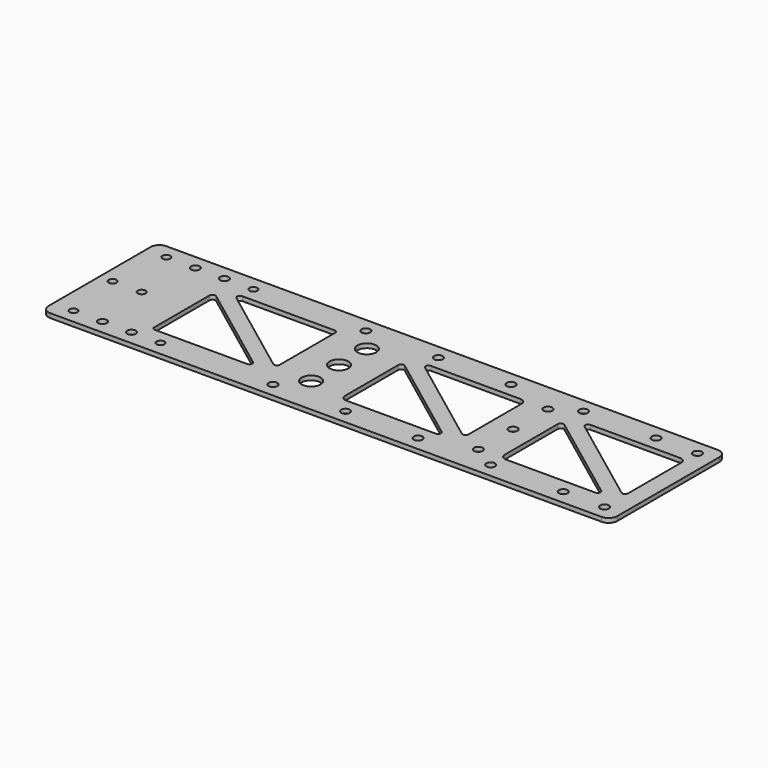
from build123d import *

# Parameters (mm, degrees)
F0_R     = 3.25
F0_R_2   = 1.35
F0_R_3   = 1.5
F1_DEPTH = 1.5


# Not quite as in the source:
# - a feature names something its author has since deleted; it is built from what else it names


with BuildPart() as f1:
    # F0 (on Top) → F1 (new body)
    with BuildSketch(Plane.XY):
        with BuildLine():
            Line((61.8890674149, 727.822291851), (-128.1109325851, 727.822291851))
            ThreePointArc((-128.1109325851, 727.822291851), (-130.2322529287, 726.9436121946), (-131.1109325851, 724.822291851))
            Line((-131.1109325851, 724.822291851), (-131.1109325851, 702.822291851))
            Line((-131.1109325851, 702.822291851), (-127.9609325851, 702.822291851))
            ThreePointArc((-127.9609325851, 702.822291851), (-126.6109325851, 704.172291851), (-125.2609325851, 702.822291851))
            Line((-125.2609325851, 702.822291851), (-117.9609325851, 702.822291851))
            ThreePointArc((-117.9609325851, 702.822291851), (-116.6109325851, 704.172291851), (-115.2609325851, 702.822291851))
            Line((-115.2609325851, 702.822291851), (-101.1109325851, 702.822291851))
            Line((-101.1109325851, 702.822291851), (-101.1109325851, 712.697291851))
            Line((-101.1109325851, 712.697291851), (-101.1109325851, 714.697291851))
            Line((-101.1109325851, 714.697291851), (-101.1109325851, 714.822291851))
            ThreePointArc((-101.1109325851, 714.822291851), (-100.8472193445, 716.0522246827), (-100.1024427382, 717.0659244658))
            ThreePointArc((-100.1024427382, 717.0659244658), (-99.1760856623, 717.6268326195), (-98.1109325851, 717.822291851))
            Line((-98.1109325851, 717.822291851), (-96.9442659185, 717.822291851))
            Line((-96.9442659185, 717.822291851), (-93.9442659185, 717.822291851))
            Line((-93.9442659185, 717.822291851), (-62.1109325851, 717.822291851))
            ThreePointArc((-62.1109325851, 717.822291851), (-61.403825804, 717.5293986322), (-61.1109325851, 716.822291851))
            Line((-61.1109325851, 716.822291851), (-61.1109325851, 702.822291851))
            Line((-61.1109325851, 702.822291851), (-51.8609325851, 702.822291851))
            ThreePointArc((-51.8609325851, 702.822291851), (-48.6109325851, 706.072291851), (-45.3609325851, 702.822291851))
            Line((-45.3609325851, 702.822291851), (-36.1109325851, 702.822291851))
            Line((-36.1109325851, 702.822291851), (-36.1109325851, 712.697291851))
            Line((-36.1109325851, 712.697291851), (-36.1109325851, 714.697291851))
            Line((-36.1109325851, 714.697291851), (-36.1109325851, 715.822291851))
            ThreePointArc((-36.1109325851, 715.822291851), (-35.9351237581, 716.6422470721), (-35.4386060205, 717.3180469276))
            ThreePointArc((-35.4386060205, 717.3180469276), (-34.8210346366, 717.6919856967), (-34.1109325851, 717.822291851))
            Line((-34.1109325851, 717.822291851), (-31.9442659185, 717.822291851))
            Line((-31.9442659185, 717.822291851), (-28.9442659185, 717.822291851))
            Line((-28.9442659185, 717.822291851), (1.8890674149, 717.822291851))
            ThreePointArc((1.8890674149, 717.822291851), (3.3032809772, 717.2365054134), (3.8890674149, 715.822291851))
            Line((3.8890674149, 715.822291851), (3.8890674149, 702.822291851))
            Line((3.8890674149, 702.822291851), (9.8890674149, 702.822291851))
            ThreePointArc((9.8890674149, 702.822291851), (11.3890674149, 704.322291851), (12.8890674149, 702.822291851))
            Line((12.8890674149, 702.822291851), (18.8890674149, 702.822291851))
            Line((18.8890674149, 702.822291851), (18.8890674149, 712.697291851))
            Line((18.8890674149, 712.697291851), (18.8890674149, 714.697291851))
            Line((18.8890674149, 714.697291851), (18.8890674149, 715.822291851))
            ThreePointArc((18.8890674149, 715.822291851), (19.0648762419, 716.6422470721), (19.5613939795, 717.3180469276))
            ThreePointArc((19.5613939795, 717.3180469276), (20.1789653634, 717.6919856967), (20.8890674149, 717.822291851))
            Line((20.8890674149, 717.822291851), (23.0557340815, 717.822291851))
            Line((23.0557340815, 717.822291851), (26.0557340815, 717.822291851))
            Line((26.0557340815, 717.822291851), (56.8890674149, 717.822291851))
            ThreePointArc((56.8890674149, 717.822291851), (58.3032809772, 717.2365054134), (58.8890674149, 715.822291851))
            Line((58.8890674149, 715.822291851), (58.8890674149, 702.822291851))
            Line((58.8890674149, 702.822291851), (64.8890674149, 702.822291851))
            Line((64.8890674149, 702.822291851), (64.8890674149, 724.822291851))
            ThreePointArc((64.8890674149, 724.822291851), (64.0103877584, 726.9436121946), (61.8890674149, 727.822291851))
        make_face()
        with Locations((-48.6109325851, 714.822291851)):
            Circle(F0_R, mode=Mode.SUBTRACT)
        with Locations((-124.1109325851, 722.822291851)):
            Circle(F0_R_2, mode=Mode.SUBTRACT)
        with Locations((-114.1109325851, 722.822291851)):
            Circle(F0_R_3, mode=Mode.SUBTRACT)
        with Locations((-104.1109325851, 722.822291851)):
            Circle(F0_R_3, mode=Mode.SUBTRACT)
        with Locations((-94.1109325851, 722.822291851)):
            Circle(F0_R_2, mode=Mode.SUBTRACT)
        with Locations((-55.3609325851, 722.822291851)):
            Circle(F0_R_3, mode=Mode.SUBTRACT)
        with Locations((11.3890674149, 717.822291851)):
            Circle(F0_R_3, mode=Mode.SUBTRACT)
        with Locations((-30.3609325851, 722.822291851)):
            Circle(F0_R_3, mode=Mode.SUBTRACT)
        with Locations((-5.3609325851, 722.822291851)):
            Circle(F0_R_3, mode=Mode.SUBTRACT)
        with Locations((19.6390674149, 722.822291851)):
            Circle(F0_R_3, mode=Mode.SUBTRACT)
        with Locations((23.8890674149, 722.822291851)):
            Circle(F0_R_3, mode=Mode.SUBTRACT)
        with Locations((44.6390674149, 722.822291851)):
            Circle(F0_R_3, mode=Mode.SUBTRACT)
        with Locations((58.8890674149, 722.822291851)):
            Circle(F0_R_3, mode=Mode.SUBTRACT)
        with BuildLine():
            Line((-127.9609325851, 702.822291851), (-131.1109325851, 702.822291851))
            Line((-131.1109325851, 702.822291851), (-131.1109325851, 680.822291851))
            ThreePointArc((-131.1109325851, 680.822291851), (-130.2322529287, 678.7009715075), (-128.1109325851, 677.822291851))
            Line((-128.1109325851, 677.822291851), (61.8890674149, 677.822291851))
            ThreePointArc((61.8890674149, 677.822291851), (64.0103877584, 678.7009715075), (64.8890674149, 680.822291851))
            Line((64.8890674149, 680.822291851), (64.8890674149, 702.822291851))
            Line((64.8890674149, 702.822291851), (58.8890674149, 702.822291851))
            Line((58.8890674149, 702.822291851), (58.8890674149, 692.947291851))
            Line((58.8890674149, 692.947291851), (58.8890674149, 690.947291851))
            Line((58.8890674149, 690.947291851), (58.8890674149, 689.822291851))
            ThreePointArc((58.8890674149, 689.822291851), (58.7132585878, 689.0023366299), (58.2167408502, 688.3265367745))
            ThreePointArc((58.2167408502, 688.3265367745), (57.5991694663, 687.9525980054), (56.8890674149, 687.822291851))
            Line((56.8890674149, 687.822291851), (54.7224007482, 687.822291851))
            Line((54.7224007482, 687.822291851), (51.7224007482, 687.822291851))
            Line((51.7224007482, 687.822291851), (20.8890674149, 687.822291851))
            ThreePointArc((20.8890674149, 687.822291851), (19.4748538525, 688.4080782887), (18.8890674149, 689.822291851))
            Line((18.8890674149, 689.822291851), (18.8890674149, 702.822291851))
            Line((18.8890674149, 702.822291851), (12.8890674149, 702.822291851))
            ThreePointArc((12.8890674149, 702.822291851), (11.3890674149, 701.322291851), (9.8890674149, 702.822291851))
            Line((9.8890674149, 702.822291851), (3.8890674149, 702.822291851))
            Line((3.8890674149, 702.822291851), (3.8890674149, 692.947291851))
            Line((3.8890674149, 692.947291851), (3.8890674149, 690.947291851))
            Line((3.8890674149, 690.947291851), (3.8890674149, 689.822291851))
            ThreePointArc((3.8890674149, 689.822291851), (3.7132585878, 689.0023366299), (3.2167408502, 688.3265367745))
            ThreePointArc((3.2167408502, 688.3265367745), (2.5991694663, 687.9525980054), (1.8890674149, 687.822291851))
            Line((1.8890674149, 687.822291851), (-0.2775992518, 687.822291851))
            Line((-0.2775992518, 687.822291851), (-3.2775992518, 687.822291851))
            Line((-3.2775992518, 687.822291851), (-34.1109325851, 687.822291851))
            ThreePointArc((-34.1109325851, 687.822291851), (-35.5251461475, 688.4080782887), (-36.1109325851, 689.822291851))
            Line((-36.1109325851, 689.822291851), (-36.1109325851, 702.822291851))
            Line((-36.1109325851, 702.822291851), (-45.3609325851, 702.822291851))
            ThreePointArc((-45.3609325851, 702.822291851), (-48.6109325851, 699.572291851), (-51.8609325851, 702.822291851))
            Line((-51.8609325851, 702.822291851), (-61.1109325851, 702.822291851))
            Line((-61.1109325851, 702.822291851), (-61.1109325851, 692.947291851))
            Line((-61.1109325851, 692.947291851), (-61.1109325851, 690.947291851))
            Line((-61.1109325851, 690.947291851), (-61.1109325851, 690.822291851))
            ThreePointArc((-61.1109325851, 690.822291851), (-61.3746458258, 689.5923590194), (-62.1194224321, 688.5786592362))
            ThreePointArc((-62.1194224321, 688.5786592362), (-63.045779508, 688.0177510825), (-64.1109325851, 687.822291851))
            Line((-64.1109325851, 687.822291851), (-65.2775992518, 687.822291851))
            Line((-65.2775992518, 687.822291851), (-68.2775992518, 687.822291851))
            Line((-68.2775992518, 687.822291851), (-100.1109325851, 687.822291851))
            ThreePointArc((-100.1109325851, 687.822291851), (-100.8180393663, 688.1151850699), (-101.1109325851, 688.822291851))
            Line((-101.1109325851, 688.822291851), (-101.1109325851, 702.822291851))
            Line((-101.1109325851, 702.822291851), (-115.2609325851, 702.822291851))
            ThreePointArc((-115.2609325851, 702.822291851), (-116.6109325851, 701.472291851), (-117.9609325851, 702.822291851))
            Line((-117.9609325851, 702.822291851), (-125.2609325851, 702.822291851))
            ThreePointArc((-125.2609325851, 702.822291851), (-126.6109325851, 701.472291851), (-127.9609325851, 702.822291851))
        make_face()
        with Locations((-124.1109325851, 682.822291851)):
            Circle(F0_R_2, mode=Mode.SUBTRACT)
        with Locations((-114.1109325851, 682.822291851)):
            Circle(F0_R_3, mode=Mode.SUBTRACT)
        with Locations((-104.1109325851, 682.822291851)):
            Circle(F0_R_3, mode=Mode.SUBTRACT)
        with Locations((-94.1109325851, 682.822291851)):
            Circle(F0_R_2, mode=Mode.SUBTRACT)
        with Locations((-55.3609325851, 682.822291851)):
            Circle(F0_R_3, mode=Mode.SUBTRACT)
        with Locations((-48.6109325851, 690.822291851)):
            Circle(F0_R, mode=Mode.SUBTRACT)
        with Locations((-30.3609325851, 682.822291851)):
            Circle(F0_R_3, mode=Mode.SUBTRACT)
        with Locations((-5.3609325851, 682.822291851)):
            Circle(F0_R_3, mode=Mode.SUBTRACT)
        with Locations((11.3890674149, 687.822291851)):
            Circle(F0_R_3, mode=Mode.SUBTRACT)
        with Locations((19.6390674149, 682.822291851)):
            Circle(F0_R_3, mode=Mode.SUBTRACT)
        with Locations((23.8890674149, 682.822291851)):
            Circle(F0_R_3, mode=Mode.SUBTRACT)
        with Locations((44.6390674149, 682.822291851)):
            Circle(F0_R_3, mode=Mode.SUBTRACT)
        with Locations((58.8890674149, 682.822291851)):
            Circle(F0_R_3, mode=Mode.SUBTRACT)
        with Locations((23.8890674149, 722.822291851)):
            Circle(F0_R_3)
        with Locations((23.8890674149, 682.822291851)):
            Circle(F0_R_3)
        with BuildLine():
            Line((-99.5109326053, 713.4972918661), (-85.2775992518, 702.822291851))
            Line((-85.2775992518, 702.822291851), (-81.1109325851, 702.822291851))
            Line((-81.1109325851, 702.822291851), (-100.1024427382, 717.0659244658))
            ThreePointArc((-100.1024427382, 717.0659244658), (-100.8472193445, 716.0522246827), (-101.1109325851, 714.822291851))
            Line((-101.1109325851, 714.822291851), (-101.1109325851, 714.697291851))
            Line((-101.1109325851, 714.697291851), (-99.5109326053, 713.4972918661))
        make_face()
        with BuildLine():
            Line((-100.1024427382, 717.0659244658), (-81.1109325851, 702.822291851))
            Line((-81.1109325851, 702.822291851), (-76.9442659185, 702.822291851))
            Line((-76.9442659185, 702.822291851), (-94.5442658047, 716.0222917657))
            Line((-94.5442658047, 716.0222917657), (-96.9442659185, 717.822291851))
            Line((-96.9442659185, 717.822291851), (-98.1109325851, 717.822291851))
            ThreePointArc((-98.1109325851, 717.822291851), (-99.1760856623, 717.6268326195), (-100.1024427382, 717.0659244658))
        make_face()
        with BuildLine():
            Line((-76.9442659185, 702.822291851), (-81.1109325851, 702.822291851))
            Line((-81.1109325851, 702.822291851), (-62.1194224321, 688.5786592362))
            ThreePointArc((-62.1194224321, 688.5786592362), (-61.3746458258, 689.5923590194), (-61.1109325851, 690.822291851))
            Line((-61.1109325851, 690.822291851), (-61.1109325851, 690.947291851))
            Line((-61.1109325851, 690.947291851), (-62.7109326177, 692.1472918754))
            Line((-62.7109326177, 692.1472918754), (-76.9442659185, 702.822291851))
        make_face()
        with BuildLine():
            Line((-81.1109325851, 702.822291851), (-85.2775992518, 702.822291851))
            Line((-85.2775992518, 702.822291851), (-67.6775992141, 689.6222918227))
            Line((-67.6775992141, 689.6222918227), (-65.2775992518, 687.822291851))
            Line((-65.2775992518, 687.822291851), (-64.1109325851, 687.822291851))
            ThreePointArc((-64.1109325851, 687.822291851), (-63.045779508, 688.0177510825), (-62.1194224321, 688.5786592362))
            Line((-62.1194224321, 688.5786592362), (-81.1109325851, 702.822291851))
        make_face()
        with BuildLine():
            Line((-65.2775992518, 687.822291851), (-67.6775992141, 689.6222918227))
            ThreePointArc((-67.6775992141, 689.6222918227), (-67.3831720503, 689.2695054254), (-67.2775992518, 688.822291851))
            ThreePointArc((-67.2775992518, 688.822291851), (-67.5704924706, 688.1151850699), (-68.2775992518, 687.822291851))
            Line((-68.2775992518, 687.822291851), (-65.2775992518, 687.822291851))
        make_face()
        with BuildLine():
            Line((-96.9442659185, 717.822291851), (-94.5442658047, 716.0222917657))
            ThreePointArc((-94.5442658047, 716.0222917657), (-94.892949239, 717.1385195496), (-93.9442659185, 717.822291851))
            Line((-93.9442659185, 717.822291851), (-96.9442659185, 717.822291851))
        make_face()
        with BuildLine():
            Line((-16.1109325851, 702.822291851), (-11.9442659185, 702.822291851))
            Line((-11.9442659185, 702.822291851), (-29.5442658782, 716.0222918209))
            Line((-29.5442658782, 716.0222918209), (-31.9442659185, 717.822291851))
            Line((-31.9442659185, 717.822291851), (-34.1109325851, 717.822291851))
            ThreePointArc((-34.1109325851, 717.822291851), (-34.8210346366, 717.6919856967), (-35.4386060205, 717.3180469276))
            Line((-35.4386060205, 717.3180469276), (-16.1109325851, 702.822291851))
        make_face()
        with BuildLine():
            Line((-20.2775992518, 702.822291851), (-16.1109325851, 702.822291851))
            Line((-16.1109325851, 702.822291851), (-35.4386060205, 717.3180469276))
            ThreePointArc((-35.4386060205, 717.3180469276), (-35.9351237581, 716.6422470721), (-36.1109325851, 715.822291851))
            Line((-36.1109325851, 715.822291851), (-36.1109325851, 714.697291851))
            Line((-36.1109325851, 714.697291851), (-34.5109326989, 713.4972919364))
            Line((-34.5109326989, 713.4972919364), (-20.2775992518, 702.822291851))
        make_face()
        with BuildLine():
            Line((3.2167408502, 688.3265367745), (-16.1109325851, 702.822291851))
            Line((-16.1109325851, 702.822291851), (-20.2775992518, 702.822291851))
            Line((-20.2775992518, 702.822291851), (-2.6775993691, 689.622291939))
            Line((-2.6775993691, 689.622291939), (-0.2775992518, 687.822291851))
            Line((-0.2775992518, 687.822291851), (1.8890674149, 687.822291851))
            ThreePointArc((1.8890674149, 687.822291851), (2.5991694663, 687.9525980054), (3.2167408502, 688.3265367745))
        make_face()
        with BuildLine():
            Line((2.2890673807, 692.1472918767), (-11.9442659185, 702.822291851))
            Line((-11.9442659185, 702.822291851), (-16.1109325851, 702.822291851))
            Line((-16.1109325851, 702.822291851), (3.2167408502, 688.3265367745))
            ThreePointArc((3.2167408502, 688.3265367745), (3.7132585878, 689.0023366299), (3.8890674149, 689.822291851))
            Line((3.8890674149, 689.822291851), (3.8890674149, 690.947291851))
            Line((3.8890674149, 690.947291851), (2.2890673807, 692.1472918767))
        make_face()
        with BuildLine():
            Line((-0.2775992518, 687.822291851), (-2.6775993691, 689.622291939))
            ThreePointArc((-2.6775993691, 689.622291939), (-2.3831720936, 689.2695055121), (-2.2775992518, 688.822291851))
            ThreePointArc((-2.2775992518, 688.822291851), (-2.5704924706, 688.1151850699), (-3.2775992518, 687.822291851))
            Line((-3.2775992518, 687.822291851), (-0.2775992518, 687.822291851))
        make_face()
        with BuildLine():
            Line((3.8890674149, 690.947291851), (3.8890674149, 692.947291851))
            ThreePointArc((3.8890674149, 692.947291851), (3.3362809913, 692.0528646505), (2.2890673807, 692.1472918767))
            Line((2.2890673807, 692.1472918767), (3.8890674149, 690.947291851))
        make_face()
        with BuildLine():
            Line((-31.9442659185, 717.822291851), (-29.5442658782, 716.0222918209))
            ThreePointArc((-29.5442658782, 716.0222918209), (-29.8929492245, 717.1385195932), (-28.9442659185, 717.822291851))
            Line((-28.9442659185, 717.822291851), (-31.9442659185, 717.822291851))
        make_face()
        with BuildLine():
            ThreePointArc((-36.1109325851, 712.697291851), (-35.5581462443, 713.5917190102), (-34.5109326989, 713.4972919364))
            Line((-34.5109326989, 713.4972919364), (-36.1109325851, 714.697291851))
            Line((-36.1109325851, 714.697291851), (-36.1109325851, 712.697291851))
        make_face()
        with BuildLine():
            Line((34.7224007482, 702.822291851), (38.8890674149, 702.822291851))
            Line((38.8890674149, 702.822291851), (19.5613939795, 717.3180469276))
            ThreePointArc((19.5613939795, 717.3180469276), (19.0648762419, 716.6422470721), (18.8890674149, 715.822291851))
            Line((18.8890674149, 715.822291851), (18.8890674149, 714.697291851))
            Line((18.8890674149, 714.697291851), (20.4890673011, 713.4972919364))
            Line((20.4890673011, 713.4972919364), (34.7224007482, 702.822291851))
        make_face()
        with BuildLine():
            Line((38.8890674149, 702.822291851), (43.0557340815, 702.822291851))
            Line((43.0557340815, 702.822291851), (25.4557339533, 716.0222919472))
            Line((25.4557339533, 716.0222919472), (23.0557340815, 717.822291851))
            Line((23.0557340815, 717.822291851), (20.8890674149, 717.822291851))
            ThreePointArc((20.8890674149, 717.822291851), (20.1789653634, 717.6919856967), (19.5613939795, 717.3180469276))
            Line((19.5613939795, 717.3180469276), (38.8890674149, 702.822291851))
        make_face()
        with BuildLine():
            Line((58.2167408502, 688.3265367745), (38.8890674149, 702.822291851))
            Line((38.8890674149, 702.822291851), (34.7224007482, 702.822291851))
            Line((34.7224007482, 702.822291851), (52.3224007859, 689.6222918227))
            Line((52.3224007859, 689.6222918227), (54.7224007482, 687.822291851))
            Line((54.7224007482, 687.822291851), (56.8890674149, 687.822291851))
            ThreePointArc((56.8890674149, 687.822291851), (57.5991694663, 687.9525980054), (58.2167408502, 688.3265367745))
        make_face()
        with BuildLine():
            Line((57.2890672834, 692.1472919496), (43.0557340815, 702.822291851))
            Line((43.0557340815, 702.822291851), (38.8890674149, 702.822291851))
            Line((38.8890674149, 702.822291851), (58.2167408502, 688.3265367745))
            ThreePointArc((58.2167408502, 688.3265367745), (58.7132585878, 689.0023366299), (58.8890674149, 689.822291851))
            Line((58.8890674149, 689.822291851), (58.8890674149, 690.947291851))
            Line((58.8890674149, 690.947291851), (57.2890672834, 692.1472919496))
        make_face()
        with BuildLine():
            Line((23.0557340815, 717.822291851), (25.4557339533, 716.0222919472))
            ThreePointArc((25.4557339533, 716.0222919472), (25.1070508088, 717.1385196931), (26.0557340815, 717.822291851))
            Line((26.0557340815, 717.822291851), (23.0557340815, 717.822291851))
        make_face()
        with BuildLine():
            ThreePointArc((18.8890674149, 712.697291851), (19.4418537557, 713.5917190102), (20.4890673011, 713.4972919364))
            Line((20.4890673011, 713.4972919364), (18.8890674149, 714.697291851))
            Line((18.8890674149, 714.697291851), (18.8890674149, 712.697291851))
        make_face()
        with BuildLine():
            Line((58.8890674149, 690.947291851), (58.8890674149, 692.947291851))
            ThreePointArc((58.8890674149, 692.947291851), (58.3362809369, 692.0528646233), (57.2890672834, 692.1472919496))
            Line((57.2890672834, 692.1472919496), (58.8890674149, 690.947291851))
        make_face()
        with BuildLine():
            Line((54.7224007482, 687.822291851), (52.3224007859, 689.6222918227))
            ThreePointArc((52.3224007859, 689.6222918227), (52.6168279497, 689.2695054254), (52.7224007482, 688.822291851))
            ThreePointArc((52.7224007482, 688.822291851), (52.4295075294, 688.1151850699), (51.7224007482, 687.822291851))
            Line((51.7224007482, 687.822291851), (54.7224007482, 687.822291851))
        make_face()
        with BuildLine():
            ThreePointArc((-61.1109325851, 692.947291851), (-61.6637190078, 692.052864651), (-62.7109326177, 692.1472918754))
            Line((-62.7109326177, 692.1472918754), (-61.1109325851, 690.947291851))
            Line((-61.1109325851, 690.947291851), (-61.1109325851, 692.947291851))
        make_face()
        with BuildLine():
            Line((-101.1109325851, 714.697291851), (-101.1109325851, 712.697291851))
            ThreePointArc((-101.1109325851, 712.697291851), (-100.5581461919, 713.5917190364), (-99.5109326053, 713.4972918661))
            Line((-99.5109326053, 713.4972918661), (-101.1109325851, 714.697291851))
        make_face()
    extrude(amount=F1_DEPTH)


solid = f1.part
